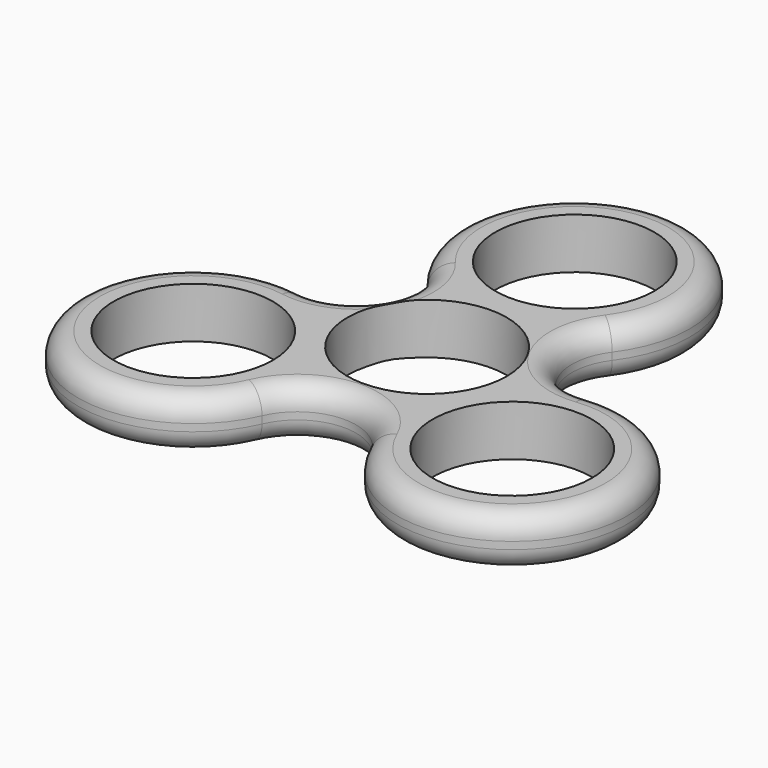
from build123d import *

# Parameters (mm, degrees)
F0_R         = 10.9855
F1_DEPTH     = 7
F2_T3_ANGLE  = 256.3995561368
F2_T6_ANGLE  = 256.0217037288
F2_T9_ANGLE  = 252.9127531636
F2_T12_ANGLE = 132.9933300565
F2_T15_ANGLE = 133.0613909212
F2_T18_ANGLE = 139.2792920515
F3_T2_ANGLE  = 256.3995561368
F3_T4_ANGLE  = 252.9127531636
F3_T6_ANGLE  = 256.0217037288
F3_T8_ANGLE  = 133.0613909212
F3_T10_ANGLE = 139.2792920515
F3_T12_ANGLE = 132.9933300565


# Not quite as in the source:
# - a fillet or chamfer that OpenCascade refuses, or shapes differently, is made with other operations: its cross-section is extruded or revolved along the edge and cut away or added
# - a feature names something its author has since deleted; it is built from what else it names


with BuildPart() as f1:
    # F0 (on Top) → F1 (new body)
    with BuildSketch(Plane.XY):
        with BuildLine():
            ThreePointArc((20.233408665, 2.951924091), (12.2068374294, 7.0151023416), (12.7372395679, 15.9958560332))
            ThreePointArc((12.7372395679, 15.9958560332), (-0.4306472142, 41.3401577589), (-12.2046104843, 15.3189998066))
            ThreePointArc((-12.2046104843, 15.3189998066), (-11.4501444105, 6.5802412239), (-19.3804348229, 2.8324932871))
            ThreePointArc((-19.3804348229, 2.8324932871), (-35.9605045031, -20.3950847915), (-7.4494474677, -19.1546329687))
            ThreePointArc((-7.4494474677, -19.1546329687), (0, -14.2708711815), (7.4494474677, -19.1546329687))
            ThreePointArc((7.4494474677, -19.1546329687), (35.7499761764, -20.7708093962), (20.233408665, 2.951924091))
        make_face()
        with Locations((-22.0074076702, -12.8236441247)):
            Circle(F0_R, mode=Mode.SUBTRACT)
        with Locations((22.0074076702, -12.8236441247)):
            Circle(F0_R, mode=Mode.SUBTRACT)
        Circle(F0_R, mode=Mode.SUBTRACT)
        with Locations((0, 25.471)):
            Circle(F0_R, mode=Mode.SUBTRACT)
    extrude(amount=F1_DEPTH)

    # F2: fillet of radius 3 on 3 edges, made by hand


with BuildPart() as f2_tool1:
    # F2_s2 → F2_t3 (revolve)
    with BuildSketch(Plane(origin=(12.1977481645, 16.3971799378, 0), x_dir=(0, 0, 1), z_dir=(-0.5968594625, -0.8023457996, 0))):
        with BuildLine():
            ThreePointArc((4, -0.6723926313), (6.1213203436, 0.2062870251), (7, 2.3276073687))
            Line((7, 2.3276073687), (7, -0.6723926313))
            Line((7, -0.6723926313), (4, -0.6723926313))
        make_face()
    revolve(axis=Axis((0, 25.471, 7), (0, 0, 1)), revolution_arc=F2_T3_ANGLE)


with BuildPart() as f2_tool4:
    # F2_s5 → F2_t6 (revolve)
    with BuildSketch(Plane(origin=(-19.3119921223, 3.2403956096, 0), x_dir=(0, 0, 1), z_dir=(0.9862133803, -0.1654786046, 0))):
        with BuildLine():
            ThreePointArc((4, 0.4136045308), (6.1213203436, 1.2922841872), (7, 3.4136045308))
            Line((7, 3.4136045308), (7, 0.4136045308))
            Line((7, 0.4136045308), (4, 0.4136045308))
        make_face()
    revolve(axis=Axis((-22.0074076702, -12.8236441247, 7), (0, 0, 1)), revolution_arc=F2_T6_ANGLE)


with BuildPart() as f2_tool7:
    # F2_s8 → F2_t9 (revolve)
    with BuildSketch(Plane(origin=(8.189951579, -18.8326013653, 0), x_dir=(0, 0, 1), z_dir=(-0.3988024469, 0.9170368631, 0))):
        with BuildLine():
            ThreePointArc((4, -0.8074965588), (6.1213203436, 0.0711830977), (7, 2.1925034412))
            Line((7, 2.1925034412), (7, -0.8074965588))
            Line((7, -0.8074965588), (4, -0.8074965588))
        make_face()
    revolve(axis=Axis((22.0074076702, -12.8236441247, 7), (0, 0, 1)), revolution_arc=F2_T9_ANGLE)


with BuildPart() as f2_tool10:
    # F2_s11 → F2_t12 (revolve)
    with BuildSketch(Plane(origin=(-8.189951579, -18.8326013653, 0), x_dir=(0, 0, 1), z_dir=(-0.3988024469, -0.9170368631, 0))):
        with BuildLine():
            ThreePointArc((4, -0.8074965588), (6.1213203436, 0.0711830977), (7, 2.1925034412))
            Line((7, 2.1925034412), (7, -0.8074965588))
            Line((7, -0.8074965588), (4, -0.8074965588))
        make_face()
    revolve(axis=Axis((0, -22.3942605097, 7), (0, 0, -1)), revolution_arc=F2_T12_ANGLE)


with BuildPart() as f2_tool13:
    # F2_s14 → F2_t15 (revolve)
    with BuildSketch(Plane(origin=(20.3085471758, 2.2837429368, 0), x_dir=(0, 0, 1), z_dir=(0.9937365805, 0.1117479688, 0))):
        with BuildLine():
            ThreePointArc((4, -0.6723926313), (6.1213203436, 0.2062870251), (7, 2.3276073687))
            Line((7, 2.3276073687), (7, -0.6723926313))
            Line((7, -0.6723926313), (4, -0.6723926313))
        make_face()
    revolve(axis=Axis((19.3170019466, 11.1012165414, 7), (0, 0, -1)), revolution_arc=F2_T15_ANGLE)


with BuildPart() as f2_tool16:
    # F2_s17 → F2_t18 (revolve)
    with BuildSketch(Plane(origin=(-12.5225873153, 15.0545013325, 0), x_dir=(0, 0, 1), z_dir=(-0.6394960752, 0.7687943612, 0))):
        with BuildLine():
            ThreePointArc((4, 0.4136045308), (6.1213203436, 1.2922841872), (7, 3.4136045308))
            Line((7, 3.4136045308), (7, 0.4136045308))
            Line((7, 0.4136045308), (4, 0.4136045308))
        make_face()
    revolve(axis=Axis((-18.1094514577, 10.4072538085, 7), (0, 0, -1)), revolution_arc=F2_T18_ANGLE)


with BuildPart() as f1_1:
    add(f1.part)

    # F2_t19: cut F2_tool1, F2_tool4, F2_tool7, F2_tool10, F2_tool13, F2_tool16
    add([f2_tool1.part, f2_tool4.part, f2_tool7.part, f2_tool10.part, f2_tool13.part, f2_tool16.part], mode=Mode.SUBTRACT)

    # F3: fillet of radius 3 on 6 edges, made by hand

    # F3_s1 → F3_t2 (revolve, cut)
    with BuildSketch(Plane(origin=(12.1977481645, 16.3971799378, 0), x_dir=(0, 0, 1), z_dir=(-0.5968594625, -0.8023457996, 0))):
        with BuildLine():
            ThreePointArc((0, 2.3276073687), (0.8786796564, 0.2062870251), (3, -0.6723926313))
            Line((3, -0.6723926313), (0, -0.6723926313))
            Line((0, -0.6723926313), (0, 2.3276073687))
        make_face()
    revolve(axis=Axis((0, 25.471, 0), (0, 0, 1)), revolution_arc=F3_T2_ANGLE, mode=Mode.SUBTRACT)

    # F3_s3 → F3_t4 (revolve, cut)
    with BuildSketch(Plane(origin=(8.189951579, -18.8326013653, 0), x_dir=(0, 0, 1), z_dir=(-0.3988024469, 0.9170368631, 0))):
        with BuildLine():
            ThreePointArc((0, 2.1925034412), (0.8786796564, 0.0711830977), (3, -0.8074965588))
            Line((3, -0.8074965588), (0, -0.8074965588))
            Line((0, -0.8074965588), (0, 2.1925034412))
        make_face()
    revolve(axis=Axis((22.0074076702, -12.8236441247, 0), (0, 0, 1)), revolution_arc=F3_T4_ANGLE, mode=Mode.SUBTRACT)

    # F3_s5 → F3_t6 (revolve, cut)
    with BuildSketch(Plane(origin=(-19.3119921223, 3.2403956096, 0), x_dir=(0, 0, 1), z_dir=(0.9862133803, -0.1654786046, 0))):
        with BuildLine():
            ThreePointArc((0, 3.4136045308), (0.8786796564, 1.2922841872), (3, 0.4136045308))
            Line((3, 0.4136045308), (0, 0.4136045308))
            Line((0, 0.4136045308), (0, 3.4136045308))
        make_face()
    revolve(axis=Axis((-22.0074076702, -12.8236441247, 0), (0, 0, 1)), revolution_arc=F3_T6_ANGLE, mode=Mode.SUBTRACT)

    # F3_s7 → F3_t8 (revolve, cut)
    with BuildSketch(Plane(origin=(20.3085471758, 2.2837429368, 0), x_dir=(0, 0, 1), z_dir=(0.9937365805, 0.1117479688, 0))):
        with BuildLine():
            ThreePointArc((3, -0.6723926313), (0.8786796564, 0.2062870251), (0, 2.3276073687))
            Line((0, 2.3276073687), (0, -0.6723926313))
            Line((0, -0.6723926313), (3, -0.6723926313))
        make_face()
    revolve(axis=Axis((19.3170019466, 11.1012165414, 0), (0, 0, -1)), revolution_arc=F3_T8_ANGLE, mode=Mode.SUBTRACT)

    # F3_s9 → F3_t10 (revolve, cut)
    with BuildSketch(Plane(origin=(-12.5225873153, 15.0545013325, 0), x_dir=(0, 0, 1), z_dir=(-0.6394960752, 0.7687943612, 0))):
        with BuildLine():
            ThreePointArc((0, 3.4136045308), (0.8786796564, 1.2922841872), (3, 0.4136045308))
            Line((3, 0.4136045308), (0, 0.4136045308))
            Line((0, 0.4136045308), (0, 3.4136045308))
        make_face()
    revolve(axis=Axis((-18.1094514577, 10.4072538085, 0), (0, 0, -1)), revolution_arc=F3_T10_ANGLE, mode=Mode.SUBTRACT)

    # F3_s11 → F3_t12 (revolve, cut)
    with BuildSketch(Plane(origin=(-8.189951579, -18.8326013653, 0), x_dir=(0, 0, 1), z_dir=(-0.3988024469, -0.9170368631, 0))):
        with BuildLine():
            ThreePointArc((0, 2.1925034412), (0.8786796564, 0.0711830977), (3, -0.8074965588))
            Line((3, -0.8074965588), (0, -0.8074965588))
            Line((0, -0.8074965588), (0, 2.1925034412))
        make_face()
    revolve(axis=Axis((0, -22.3942605097, 0), (0, 0, -1)), revolution_arc=F3_T12_ANGLE, mode=Mode.SUBTRACT)


solid = f1_1.part
